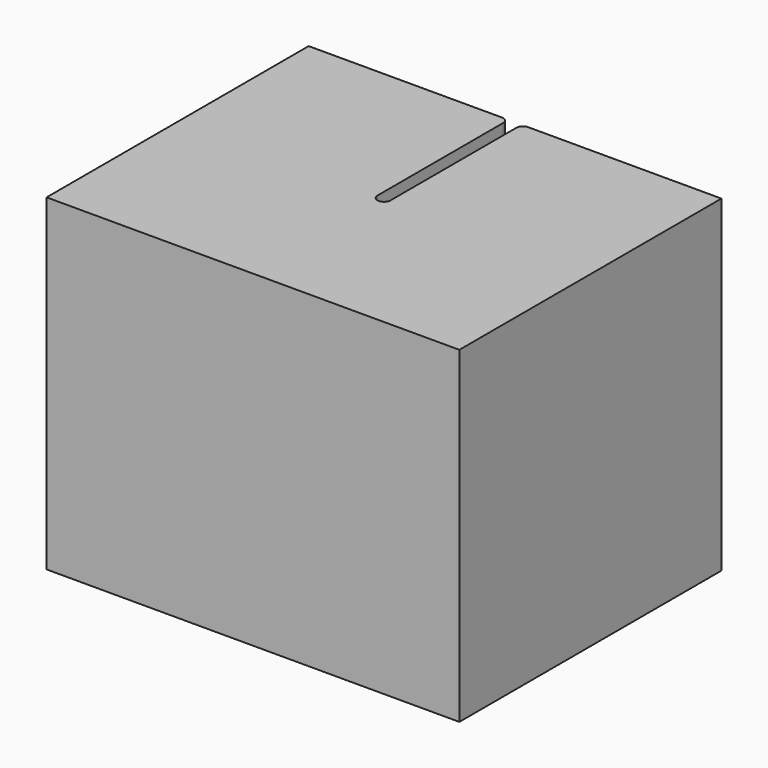
from build123d import *

# Parameters (mm, degrees)
F1_DEPTH = 10


# Not quite as in the source:
# - ends of sketch curves that miss each other by under 0.0002 mm in the source are joined


with BuildPart() as f1:
    # F0 (on Top) → F1 (new body)
    with BuildSketch(Plane.XY):
        with BuildLine():
            Line((-0.3999973293, 5), (-6.2999973293, 5))
            Line((-6.2999973293, 5), (-6.2999973293, -5))
            Line((-6.2999973293, -5), (6.3, -5))
            Line((6.3, -5), (6.3, 5))
            Line((6.3, 5), (0.4, 5))
            ThreePointArc((0.4, 5), (0.2585786438, 4.9414213562), (0.2, 4.8))
            Line((0.2, 4.8), (0.2, 0))
            ThreePointArc((0.2, 0), (0.1414213562, -0.1414213562), (0, -0.2))
            ThreePointArc((0, -0.2), (-0.1414186856, -0.1414213562), (-0.1999973293, 0))
            Line((-0.1999973293, 0), (-0.1999973293, 4.8))
            ThreePointArc((-0.1999973293, 4.8), (-0.2585759731, 4.9414213562), (-0.3999973293, 5))
        make_face()
    extrude(amount=F1_DEPTH)


solid = f1.part
